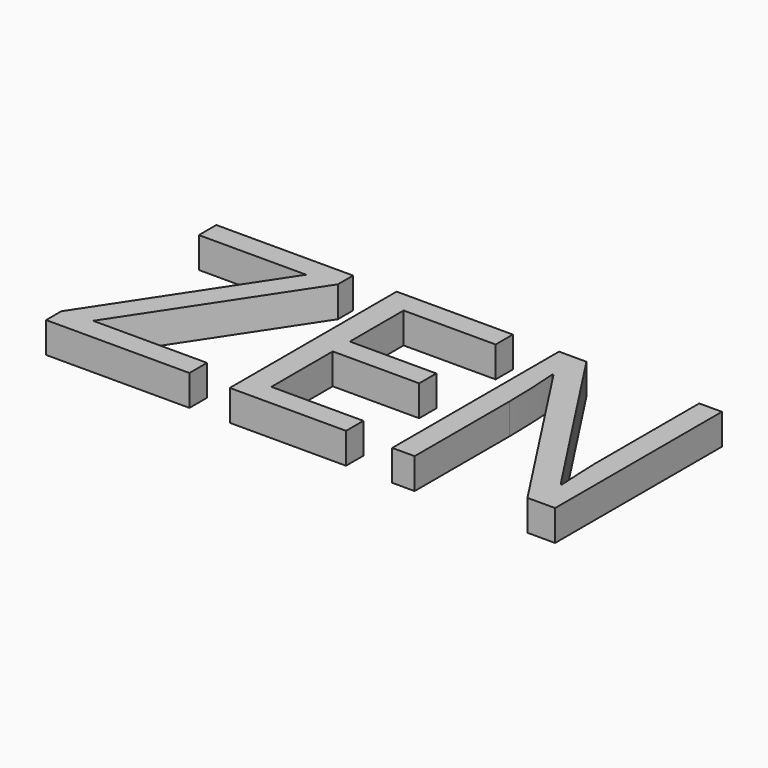
from build123d import *

# Parameters (mm, degrees)
F0_TEXT_SIZE = 120.6179356409
F1_DEPTH     = 12.7


# Not quite as in the source:
# - Text() gives the source's letters only with a copy of the font that has no kerning and outlines rounded to 1/6400 em; it was checked with that copy


with BuildPart() as f1:
    # F0 (on Top) → F1 (new body)
    with BuildSketch(Plane.XY):
        with Locations((6.8860650063, 31.8243578076)):
            Text('ZEN', F0_TEXT_SIZE, font='Open Sans', text_align=(TextAlign.LEFT, TextAlign.BOTTOM))
    extrude(amount=F1_DEPTH)


solid = f1.part
